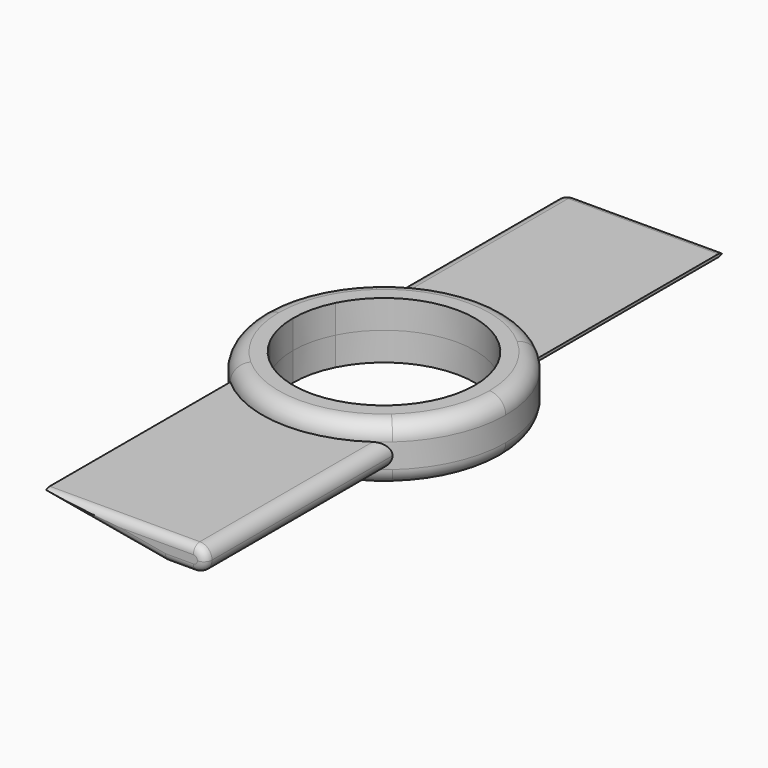
from build123d import *

# Parameters (mm, degrees)
F1_DEPTH      = 3.5
F1_DEPTH_BACK = 3.5
F2_DEPTH      = 1.5
F2_DEPTH_BACK = 1.5
F3_R          = 1.99999
F4_T4_DEPTH   = 106.7758240051
F4_S5_R       = 15
F4_T6_DEPTH   = 55
F5_R          = 1.49999
F7_T1_DEPTH   = 11.00001
F7_T3_DEPTH   = 25.2313991783
F7_T5_DEPTH   = 21.00001
F7_T7_DEPTH   = 2e-05
F7_T10_ANGLE  = 90
F7_T12_ANGLE  = 90
F8_COUNT      = 2


# Not quite as in the source:
# - a fillet or chamfer that OpenCascade refuses, or shapes differently, is made with other operations: its cross-section is extruded or revolved along the edge and cut away or added
# - a fillet or chamfer is up to 0.001 mm smaller than in the source, because OpenCascade refuses the exact size
# - a feature names something its author has since deleted; it is built from what else it names


with BuildPart() as f1:
    # F0 (on Top) → F1 (new body, two sides)
    with BuildSketch(Plane.XY) as f1_sk:
        with BuildLine():
            ThreePointArc((-10, -5.0438080852), (-11.2, 0), (-10, 5.0438080852))
            Line((-10, 5.0438080852), (-10, 11.1803398875))
            ThreePointArc((-10, 11.1803398875), (-15, 0), (-10, -11.1803398875))
            Line((-10, -11.1803398875), (-10, -5.0438080852))
        make_face()
        with BuildLine():
            ThreePointArc((-10, 5.0438080852), (0, 11.2), (10, 5.0438080852))
            Line((10, 5.0438080852), (10, 11.1803398875))
            ThreePointArc((10, 11.1803398875), (0, 15), (-10, 11.1803398875))
            Line((-10, 11.1803398875), (-10, 5.0438080852))
        make_face()
        with BuildLine():
            ThreePointArc((10, 5.0438080852), (10.8958707775, 2.5922962794), (11.2, 0))
            ThreePointArc((11.2, 0), (10.8958707775, -2.5922962794), (10, -5.0438080852))
            Line((10, -5.0438080852), (10, -11.1803398875))
            ThreePointArc((10, -11.1803398875), (13.6930639376, -6.123724357), (15, 0))
            ThreePointArc((15, 0), (13.6930639376, 6.123724357), (10, 11.1803398875))
            Line((10, 11.1803398875), (10, 5.0438080852))
        make_face()
        with BuildLine():
            Line((10, -11.1803398875), (10, -5.0438080852))
            ThreePointArc((10, -5.0438080852), (0, -11.2), (-10, -5.0438080852))
            Line((-10, -5.0438080852), (-10, -11.1803398875))
            ThreePointArc((-10, -11.1803398875), (0, -15), (10, -11.1803398875))
        make_face()
    extrude(amount=F1_DEPTH)
    extrude(f1_sk.sketch, amount=-F1_DEPTH_BACK)

    # F0 (on Top) → F2 (join, two sides)
    with BuildSketch(Plane.XY) as f2_sk:
        with BuildLine():
            ThreePointArc((-10, 11.1803398875), (0, 15), (10, 11.1803398875))
            Line((10, 11.1803398875), (10, 40))
            Line((10, 40), (-10, 40))
            Line((-10, 40), (-10, 11.1803398875))
        make_face()
    extrude(amount=F2_DEPTH)
    extrude(f2_sk.sketch, amount=-F2_DEPTH_BACK)

    # F3 (radius 2 in the source; OpenCascade refuses exactly that, so slightly less here)
    f3_edges = [f1.edges().sort_by_distance(p)[0] for p in [
        (10, 11.18034, 3.5),
        (10, 11.18034, -3.5),
    ]]
    fillet(f3_edges, radius=F3_R)

    # F4: chamfer of 15 x 2.6449047106 on 1 edges, made by hand


with BuildPart() as f4_tool2:
    # F4_s3 → F4_t4 (new body)
    with BuildSketch(Plane.XZ.offset(27.7977420588)):
        Polygon((10, 1.1449047106), (-5, -1.5), (10, -1.5), align=None)
    extrude(amount=-F4_T4_DEPTH)

    # F4_s5 → F4_t6 (cut, symmetric)
    with BuildSketch(Plane.XY.offset(-0.2)):
        Circle(F4_S5_R)
    extrude(amount=F4_T6_DEPTH, both=True, mode=Mode.SUBTRACT)


with BuildPart() as f1_1:
    add(f1.part)

    # F4_t1: cut F4_tool2
    add(f4_tool2.part, mode=Mode.SUBTRACT)

    # F5 (radius 1.5 in the source; OpenCascade refuses exactly that, so slightly less here)
    f5_edges = [f1_1.edges().sort_by_distance(p)[0] for p in [
        (-10, 25.59017, -1.5),
        (-10, 25.59017, 1.5),
    ]]
    fillet(f5_edges, radius=F5_R)

    # F7: fillet of radius 1 on 6 edges, made by hand

    # F7_s2 → F7_t1 (cut)
    with BuildSketch(Plane.YZ.offset(-8.50001)):
        with BuildLine():
            ThreePointArc((40, -0.5), (39.7071067812, -1.2071067812), (39, -1.5))
            Line((39, -1.5), (40, -1.5))
            Line((40, -1.5), (40, -0.5))
        make_face()
    extrude(amount=F7_T1_DEPTH, mode=Mode.SUBTRACT)

    # F7_s4 → F7_t3 (cut)
    with BuildSketch(Plane(origin=(12.3562727231, 0, 2.178744262), x_dir=(0, 1, 0), z_dir=(-0.984807753, 0, -0.1736481777))):
        with BuildLine():
            ThreePointArc((40, -0.3910292588), (39.7071067812, 0.3160775224), (39, 0.6089707412))
            Line((39, 0.6089707412), (40, 0.6089707412))
            Line((40, 0.6089707412), (40, -0.3910292588))
        make_face()
    extrude(amount=F7_T3_DEPTH, mode=Mode.SUBTRACT)

    # F7_s6 → F7_t5 (cut)
    with BuildSketch(Plane.YZ.offset(-8.50001)):
        with BuildLine():
            ThreePointArc((39, 1.5), (39.7071067812, 1.2071067812), (40, 0.5))
            Line((40, 0.5), (40, 1.5))
            Line((40, 1.5), (39, 1.5))
        make_face()
    extrude(amount=F7_T5_DEPTH, mode=Mode.SUBTRACT)

    # F7_s8 → F7_t7 (cut)
    with BuildSketch(Plane.XY.offset(-1e-05)):
        with BuildLine():
            ThreePointArc((-10, 39), (-9.7071067812, 39.7071067812), (-9, 40))
            Line((-9, 40), (-10, 40))
            Line((-10, 40), (-10, 39))
        make_face()
    extrude(amount=F7_T7_DEPTH, mode=Mode.SUBTRACT)

    # F7_s9 → F7_t10 (revolve, cut)
    with BuildSketch(Plane.XY.offset(-1e-05)):
        with BuildLine():
            ThreePointArc((-9, 40), (-9.7071067812, 39.7071067812), (-10, 39))
            Line((-10, 39), (-10, 40))
            Line((-10, 40), (-9, 40))
        make_face()
    revolve(axis=Axis((-8.50001, 40, -1e-05), (0, -1, 0)), revolution_arc=F7_T10_ANGLE, mode=Mode.SUBTRACT)

    # F7_s11 → F7_t12 (revolve, cut)
    with BuildSketch(Plane.YZ.offset(-8.50001)):
        with BuildLine():
            ThreePointArc((39, 1.5), (39.7071067812, 1.2071067812), (40, 0.5))
            Line((40, 0.5), (40, 1.5))
            Line((40, 1.5), (39, 1.5))
        make_face()
    revolve(axis=Axis((-8.50001, 40, 1e-05), (0, -1, 0)), revolution_arc=F7_T12_ANGLE, mode=Mode.SUBTRACT)

    # F8: F1 ×2 about axis
    f8_axis = Axis((0, 0, -0.2721771598), (0, 0, -1))


with BuildPart() as f1_2:
    add(f1_1.part)
    for i in range(1, F8_COUNT):
        add(f1_1.part.rotate(f8_axis, i * 360 / F8_COUNT))


solid = f1_2.part
